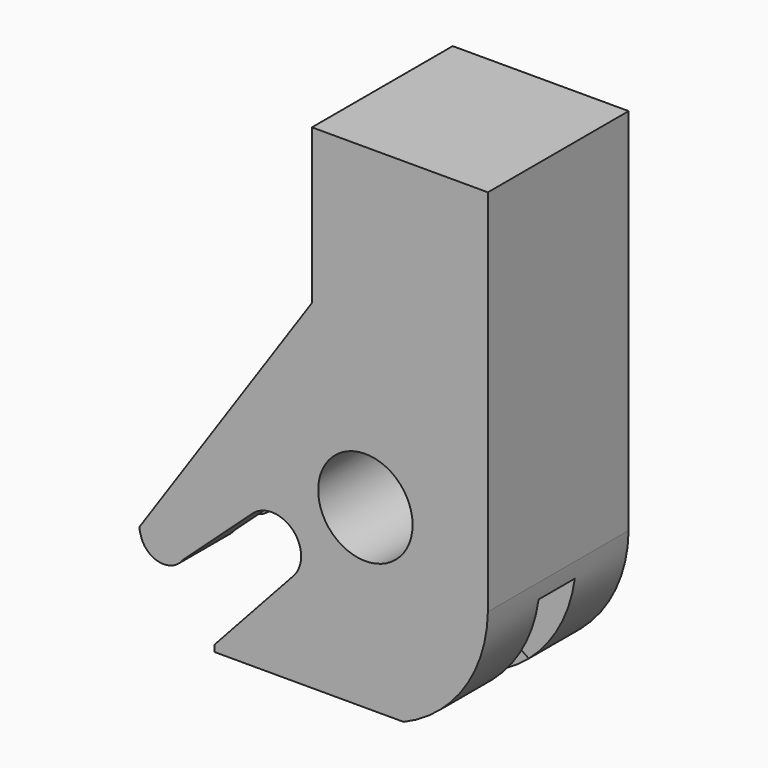
from build123d import *

# Parameters (mm, degrees)
F0_R     = 4.025
F1_DEPTH = 15
F2_W     = 4
F2_H     = 8.8454233903
F2_H_2   = 9.964544284
F3_DEPTH = 28.6711009125
F4_W     = 4
F4_H     = 9.9010998965
F5_DEPTH = 7
F7_DEPTH = 29.7172600886


# Not quite as in the source:
# - a feature names something its author has since deleted; it is built from what else it names


with BuildPart() as f1:
    # F0 (on Front) → F1 (new body)
    with BuildSketch(Plane.XZ):
        with BuildLine():
            Line((15, -11.0706584528), (15, 20))
            Line((15, 20), (0, 20))
            Line((0, 20), (0, 6.8212319165))
            Line((0, 6.8212319165), (-14.6675774532, -14.7143399477))
            ThreePointArc((-14.6675774532, -14.7143399477), (-14.7123164503, -14.8254204168), (-14.7066683885, -14.9450387593))
            Line((-14.7066683885, -14.9450387593), (-14.5789844453, -15.4207687435))
            ThreePointArc((-14.5789844453, -15.4207687435), (-13.0080916481, -16.8695228666), (-11.0253572607, -16.0724299998))
            Line((-11.0253572607, -16.0724299998), (-5.025187618, -10.5899751145))
            ThreePointArc((-5.025187618, -10.5899751145), (-1.6056896263, -10.7821354433), (-1.6008698149, -14.2070250586))
            Line((-1.6008698149, -14.2070250586), (-8.307190612, -21.5265534699))
            Line((-8.307190612, -21.5265534699), (-8.307190612, -22.085826844))
            Line((-8.307190612, -22.085826844), (7.8228749335, -22.085826844))
            ThreePointArc((7.8228749335, -22.085826844), (12.9859504737, -17.8510774103), (15, -11.4844412258))
            Line((15, -11.4844412258), (15, -11.0706584528))
        make_face()
        with Locations((4.5535718091, -7.0535713993)):
            Circle(F0_R, mode=Mode.SUBTRACT)
    extrude(amount=F1_DEPTH)

    # F2 (on face) → F3 (cut, through all)
    with BuildSketch(Plane(origin=(-3.1736560215, 0, 2.1615328257), x_dir=(0, -1, 0), z_dir=(-0.8265088883, 0, 0.5629236693))):
        with Locations((7.5, -24.8409709683)):
            Rectangle(F2_W, F2_H)
        with Locations((7.5, -15.4359871311)):
            Rectangle(F2_W, F2_H_2)
    extrude(amount=-F3_DEPTH, mode=Mode.SUBTRACT)

    # F4 (on face) → F5 (cut)
    with BuildSketch(Plane(origin=(-3.1736560215, 0, 2.1615328257), x_dir=(0, -1, 0), z_dir=(-0.8265088883, 0, 0.5629236693))):
        with Locations((7.5, -5.5031650409)):
            Rectangle(F4_W, F4_H)
    extrude(amount=-F5_DEPTH, mode=Mode.SUBTRACT)

    # F6 (on face) → F7 (cut, through all)
    with BuildSketch(Plane.YZ.offset(15)):
        Polygon((-9.4687892124, -16.3104510802), (-9.4687892124, -22.085826844), (-5.6066988036, -22.085826844), (-5.6066988036, -16.3104510802), (-5.6066988036, -12.8443576396), (-9.4687892124, -12.8443576396), align=None)
    extrude(amount=-F7_DEPTH, mode=Mode.SUBTRACT)


solid = f1.part
